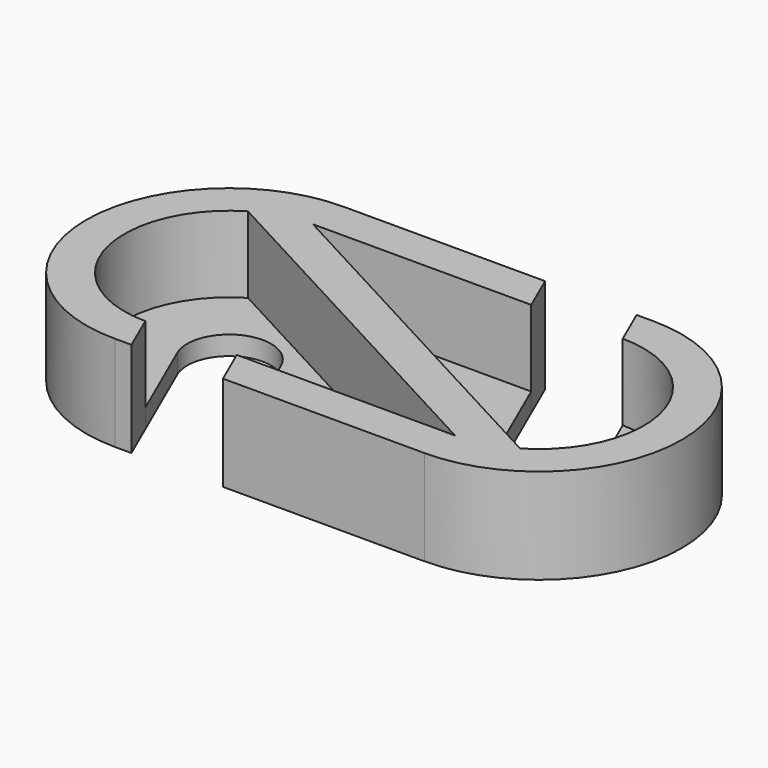
from build123d import *

# Parameters (mm, degrees)
F1_DEPTH = 4
F2_DEPTH = 0.8


# Not quite as in the source:
# - a feature names something its author has since deleted; it is built from what else it names


with BuildPart() as f1:
    # F0 (on Top) → F1 (new body)
    with BuildSketch(Plane.XY):
        with BuildLine():
            Line((8.4610678831, 6), (0, 6))
            ThreePointArc((0, 6), (-6, 0), (0, -6))
            Line((0, -6), (0.6982972488, -6))
            Line((0.6982972488, -6), (0, -4.4))
            ThreePointArc((0, -4.4), (-4.2440131224, -1.1611858666), (-2.2400400253, 3.7871124469))
            Line((-2.2400400253, 3.7871124469), (13, -4.4))
            Line((13, -4.4), (3.8406348682, -4.4))
            Line((3.8406348682, -4.4), (4.5389321169, -6))
            Line((4.5389321169, -6), (13, -6))
            ThreePointArc((13, -6), (19, 0), (13, 6))
            Line((13, 6), (12.3017027512, 6))
            Line((12.3017027512, 6), (13, 4.4))
            ThreePointArc((13, 4.4), (17.2440131224, 1.1611858666), (15.2400400253, -3.7871124469))
            Line((15.2400400253, -3.7871124469), (0, 4.4))
            Line((0, 4.4), (9.1593651318, 4.4))
            Line((9.1593651318, 4.4), (8.4610678831, 6))
        make_face()
    extrude(amount=F1_DEPTH)

    # F0 (on Top) → F2 (join)
    with BuildSketch(Plane.XY):
        with BuildLine():
            ThreePointArc((-2.2400400253, 3.7871124469), (-4.2440131224, -1.1611858666), (0, -4.4))
            Line((0, -4.4), (-0.8065333223, -2.552))
            Line((-0.8065333223, -2.552), (-1.6130666446, -0.704))
            ThreePointArc((-1.6130666446, -0.704), (-0.704, 1.6130666446), (1.6130666446, 0.704))
            Line((1.6130666446, 0.704), (3.8406348682, -4.4))
            Line((3.8406348682, -4.4), (13, -4.4))
            Line((13, -4.4), (-2.2400400253, 3.7871124469))
        make_face()
        with BuildLine():
            Line((11.3869333554, -0.704), (9.1593651318, 4.4))
            Line((9.1593651318, 4.4), (0, 4.4))
            Line((0, 4.4), (15.2400400253, -3.7871124469))
            ThreePointArc((15.2400400253, -3.7871124469), (17.2440131224, 1.1611858666), (13, 4.4))
            Line((13, 4.4), (14.6130666446, 0.704))
            ThreePointArc((14.6130666446, 0.704), (13.704, -1.6130666446), (11.3869333554, -0.704))
        make_face()
    extrude(amount=F2_DEPTH)


solid = f1.part
